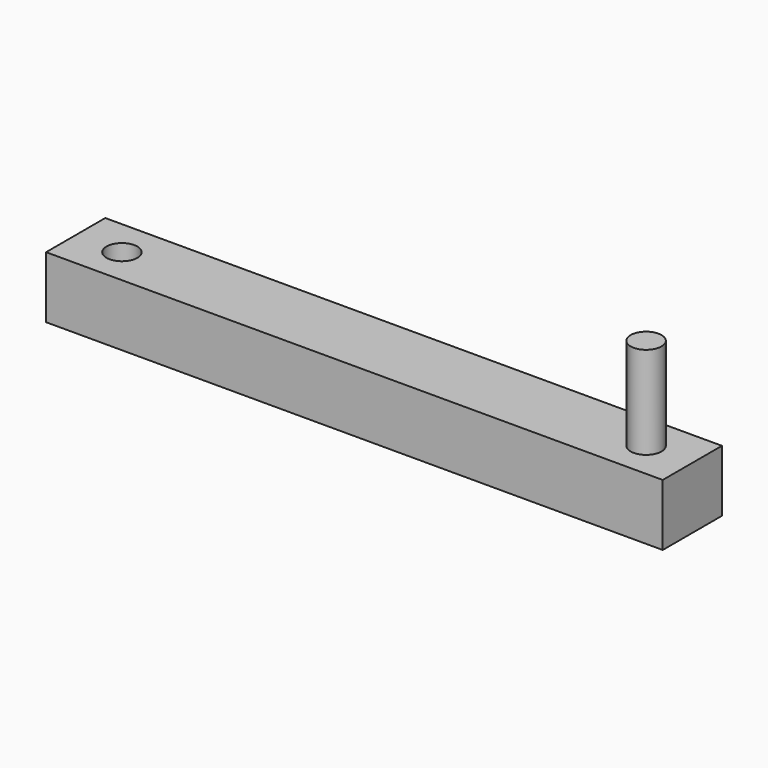
from build123d import *

# Parameters (mm, degrees)
F0_R     = 4
F0_R_2   = 2.5
F1_DEPTH = 10
F2_DEPTH = 25


with BuildPart() as f1:
    # F0 (on Top) → F1 (new body)
    with BuildSketch(Plane.XY):
        with BuildLine():
            ThreePointArc((113.5607177772, 44), (112.5, 50), (113.5607177772, 56))
            Line((113.5607177772, 56), (73.5, 56))
            Line((73.5, 56), (73.5, 44))
            Line((73.5, 44), (113.5607177772, 44))
        make_face()
        with BuildLine():
            ThreePointArc((146.4392822228, 44), (147.2327803749, 46.9534805842), (147.5, 50))
            ThreePointArc((147.5, 50), (147.2327803749, 53.0465194158), (146.4392822228, 56))
            Line((146.4392822228, 56), (113.5607177772, 56))
            ThreePointArc((113.5607177772, 56), (112.5, 50), (113.5607177772, 44))
            Line((113.5607177772, 44), (146.4392822228, 44))
        make_face()
        with Locations((130, 50)):
            Circle(F0_R, mode=Mode.SUBTRACT)
        with Locations((143, 50)):
            Circle(F0_R_2, mode=Mode.SUBTRACT)
        with BuildLine():
            Line((73.5, 44), (73.5, 56))
            Line((73.5, 56), (50.5, 56))
            Line((50.5, 56), (50.5, 52.1794494718))
            ThreePointArc((50.5, 52.1794494718), (50.8733971724, 51.1180339887), (51, 50))
            ThreePointArc((51, 50), (50.8733971724, 48.8819660113), (50.5, 47.8205505282))
            Line((50.5, 47.8205505282), (50.5, 44))
            Line((50.5, 44), (73.5, 44))
        make_face()
        with Locations((58, 50)):
            Circle(F0_R_2, mode=Mode.SUBTRACT)
        with Locations((130, 50)):
            Circle(F0_R)
        with BuildLine():
            ThreePointArc((146.4392822228, 56), (147.2327803749, 53.0465194158), (147.5, 50))
            ThreePointArc((147.5, 50), (147.2327803749, 46.9534805842), (146.4392822228, 44))
            Line((146.4392822228, 44), (150.5, 44))
            Line((150.5, 44), (150.5, 56))
            Line((150.5, 56), (146.4392822228, 56))
        make_face()
        with BuildLine():
            ThreePointArc((51, 50), (50.8733971724, 51.1180339887), (50.5, 52.1794494718))
            Line((50.5, 52.1794494718), (50.5, 47.8205505282))
            ThreePointArc((50.5, 47.8205505282), (50.8733971724, 48.8819660113), (51, 50))
        make_face()
    extrude(amount=F1_DEPTH)


with BuildPart() as f2:
    # F0 (on Top) → F2 (new body)
    with BuildSketch(Plane.XY):
        with Locations((143, 50)):
            Circle(F0_R_2)
    extrude(amount=F2_DEPTH)


solid = Compound([f1.part, f2.part])
